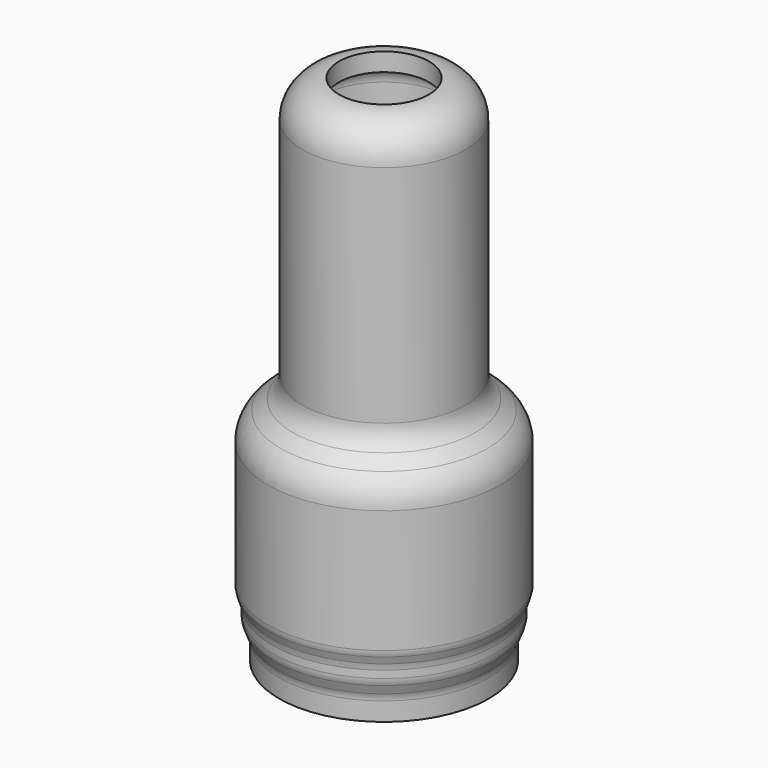
from build123d import *

# Parameters (mm, degrees)
F2_R = 12.7
F3_T = -6.35


# Not quite as in the source:
# - a shell that OpenCascade refuses in one call is made with other operations: the cavity is built on its own and cut out


with BuildPart() as f1:
    # F0 (on Front) → F1 (revolve)
    with BuildSketch(Plane.XZ):
        with BuildLine():
            Line((0, 177.8), (0, 0))
            Line((0, 0), (36.3681800663, 0))
            Line((36.3681800663, 0), (36.3681800663, 6.3854855233))
            ThreePointArc((36.3681800663, 6.3854855233), (36.4892388276, 7.6194997229), (36.847799293, 8.8064625112))
            Line((36.847799293, 8.8064625112), (38.1861001037, 12.0515719803))
            ThreePointArc((38.1861001037, 12.0515719803), (38.544660569, 13.2385347687), (38.6657193303, 14.4725489682))
            Line((38.6657193303, 14.4725489682), (38.6657193303, 16.9916158246))
            ThreePointArc((38.6657193303, 16.9916158246), (38.7581258692, 18.0709786346), (39.032656047, 19.1189272142))
            Line((39.032656047, 19.1189272142), (39.9574606684, 21.7199402117))
            ThreePointArc((39.9574606684, 21.7199402117), (40.2319908462, 22.7678887913), (40.3243973851, 23.8472516013))
            Line((40.3243973851, 23.8472516013), (40.3243973851, 66.5440567582))
            ThreePointArc((40.3243973851, 66.5440567582), (39.1467795533, 71.8849096086), (35.8323172009, 76.235292608))
            Line((35.8323172009, 76.235292608), (31.6692702472, 79.7611541302))
            ThreePointArc((31.6692702472, 79.7611541302), (29.1834234829, 83.0239413798), (28.3002101091, 87.0295810176))
            Line((28.3002101091, 87.0295810176), (28.3002101091, 177.8))
            Line((28.3002101091, 177.8), (0, 177.8))
        make_face()
    revolve(axis=Axis((0, 0, 88.9), (0, 0, -1)))

    # F2
    f2_edges = [f1.edges().sort_by_distance(p)[0] for p in [
        (-28.30021, 0, 177.8),
    ]]
    fillet(f2_edges, radius=F2_R)

    # F3: a shell. OpenCascade refuses it in one call, so the cavity is built on its own and cut out:
    # the body offset inwards by the wall thickness, plus a prism from it out through each open face.
    f3_core = offset(f1.part, amount=F3_T, kind=Kind.INTERSECTION, mode=Mode.PRIVATE)
    f3_exits = [f3_core.faces().sort_by_distance(p)[0] for p in [
        (0, 0, 171.45),
    ]]
    add(f3_core, mode=Mode.SUBTRACT)
    extrude(f3_exits, amount=-F3_T, mode=Mode.SUBTRACT)


solid = f1.part
